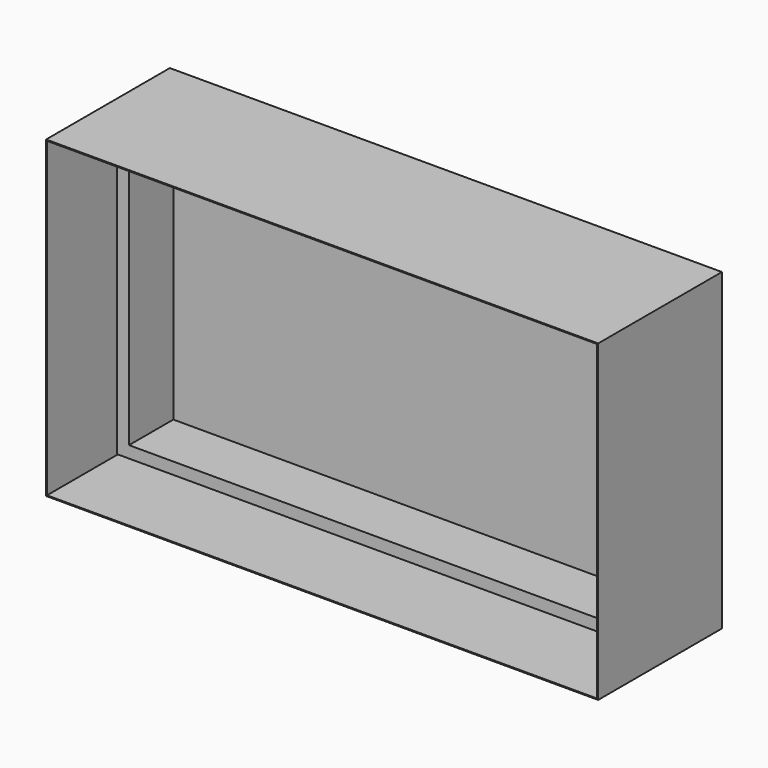
from build123d import *

# Parameters (mm, degrees)
F0_W     = 118.8842207193
F0_H     = 67.5890743732
F1_DEPTH = 33.3094447851
F2_T     = -0.2
F3_W     = 118.2425096631
F3_H     = 66.9943261892
F4_DEPTH = 14.4755076617
F5_T     = -2.54


with BuildPart() as f1:
    # F0 (on Front) → F1 (new body)
    with BuildSketch(Plane.XZ):
        Rectangle(F0_W, F0_H)
    extrude(amount=F1_DEPTH)

    # F2
    f2_openings = [f1.faces().sort_by_distance(p)[0] for p in [
        (0, -33.309445, 0),
    ]]
    offset(amount=F2_T, openings=f2_openings)

    # F3 (on Front) → F4 (join)
    with BuildSketch(Plane.XZ):
        with Locations((-0.072285533, 0.0539822504)):
            Rectangle(F3_W, F3_H)
    extrude(amount=F4_DEPTH)

    # F5
    f5_openings = [f1.faces().sort_by_distance(p)[0] for p in [
        (0, -16.754722, 33.594537),
        (-0.072286, -14.475508, 0.053982),
    ]]
    offset(amount=F5_T, openings=f5_openings)


solid = f1.part
